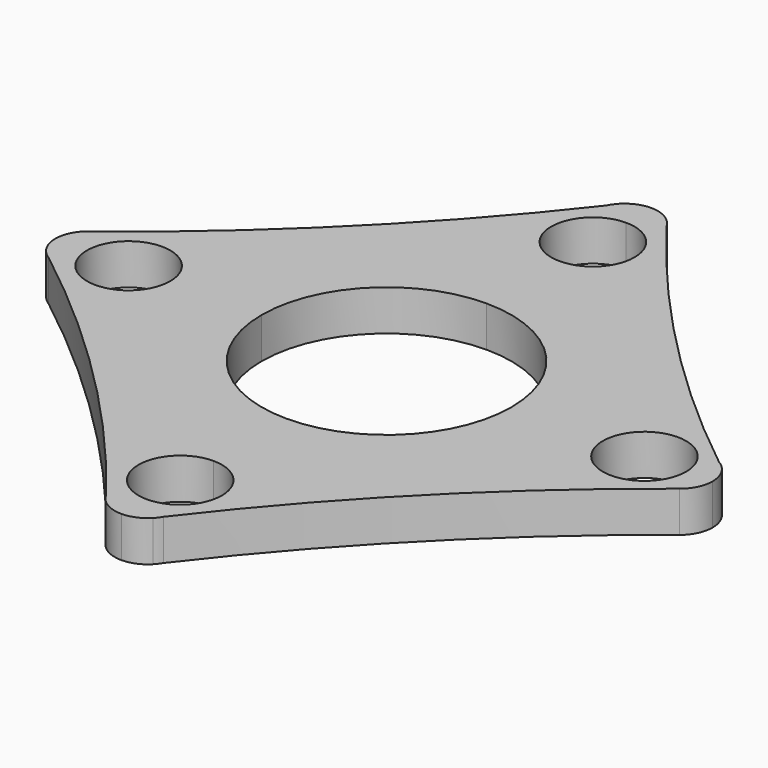
from build123d import *

# Parameters (mm, degrees)
F1_DEPTH = 1.5


with BuildPart() as f1:
    # F0 (on Top) → F1 (new body)
    with BuildSketch(Plane.XY):
        with BuildLine():
            ThreePointArc((-11.0335932724, 0), (-9.5, 1.5335932724), (-7.9664067276, 0))
            Line((-7.9664067276, 0), (-4.6, 0))
            ThreePointArc((-4.6, 0), (-3.2526911935, 3.2526911935), (0, 4.6))
            Line((0, 4.6), (0, 7.9664067276))
            ThreePointArc((0, 7.9664067276), (-1.5335932724, 9.5), (0, 11.0335932724))
            Line((0, 11.0335932724), (0, 12.2052515495))
            ThreePointArc((0, 12.2052515495), (-0.4345010394, 12.1317339839), (-0.8145803081, 11.9087188829))
            ThreePointArc((-0.8145803081, 11.9087188829), (-0.9635912872, 11.7146325201), (-1.1134019503, 11.5211627464))
            ThreePointArc((-1.1134019503, 11.5211627464), (-6.0214332546, 5.9647454006), (-11.5844815273, 1.064231252))
            ThreePointArc((-11.5844815273, 1.064231252), (-11.7185491453, 0.9605716693), (-11.8529124882, 0.8572956927))
            ThreePointArc((-11.8529124882, 0.8572956927), (-12.1114910997, 0.4629412091), (-12.2012897293, 0))
            Line((-12.2012897293, 0), (-11.0335932724, 0))
        make_face()
        with BuildLine():
            Line((-4.6, 0), (-7.9664067276, 0))
            ThreePointArc((-7.9664067276, 0), (-9.5, -1.5335932724), (-11.0335932724, 0))
            Line((-11.0335932724, 0), (-12.2012897293, 0))
            ThreePointArc((-12.2012897293, 0), (-12.1017179659, -0.4794729938), (-11.8217098669, -0.8812245989))
            ThreePointArc((-11.8217098669, -0.8812245989), (-11.721781237, -0.9580802015), (-11.6220162383, -1.0351480919))
            ThreePointArc((-11.6220162383, -1.0351480919), (-6.0202525949, -5.9659244981), (-1.0822216309, -11.5612941984))
            ThreePointArc((-1.0822216309, -11.5612941984), (-0.9646757294, -11.7132260984), (-0.8476226636, -11.8655380184))
            ThreePointArc((-0.8476226636, -11.8655380184), (-0.4559625925, -12.1137220892), (0, -12.1979305118))
            Line((0, -12.1979305118), (0, -11.0335932724))
            ThreePointArc((0, -11.0335932724), (-1.5335932724, -9.5), (0, -7.9664067276))
            Line((0, -7.9664067276), (0, -4.6))
            ThreePointArc((0, -4.6), (-3.2526911935, -3.2526911935), (-4.6, 0))
        make_face()
        with BuildLine():
            Line((0, 7.9664067276), (0, 4.6))
            ThreePointArc((0, 4.6), (3.2526911935, 3.2526911935), (4.6, 0))
            Line((4.6, 0), (7.9664067276, 0))
            ThreePointArc((7.9664067276, 0), (9.5, 1.5335932724), (11.0335932724, 0))
            Line((11.0335932724, 0), (12.0049398392, 0))
            ThreePointArc((12.0049398392, 0), (11.9193137164, 0.4573515512), (11.6687643937, 0.849432297))
            ThreePointArc((11.6687643937, 0.849432297), (11.5305346329, 0.9577272788), (11.3926261985, 1.0664311591))
            ThreePointArc((11.3926261985, 1.0664311591), (5.8870136821, 6.0076850195), (1.0395559509, 11.5960579882))
            ThreePointArc((1.0395559509, 11.5960579882), (0.9473724033, 11.7171151321), (0.8554998188, 11.838408441))
            ThreePointArc((0.8554998188, 11.838408441), (0.4640913385, 12.1065803567), (0, 12.2052515495))
            Line((0, 12.2052515495), (0, 11.0335932724))
            ThreePointArc((0, 11.0335932724), (1.0844142025, 10.5844142025), (1.5335932724, 9.5))
            ThreePointArc((1.5335932724, 9.5), (1.0844142025, 8.4155857975), (0, 7.9664067276))
        make_face()
        with BuildLine():
            ThreePointArc((4.6, 0), (3.2526911935, -3.2526911935), (0, -4.6))
            Line((0, -4.6), (0, -7.9664067276))
            ThreePointArc((0, -7.9664067276), (1.0844142025, -8.4155857975), (1.5335932724, -9.5))
            ThreePointArc((1.5335932724, -9.5), (1.0844142025, -10.5844142025), (0, -11.0335932724))
            Line((0, -11.0335932724), (0, -12.1979305118))
            ThreePointArc((0, -12.1979305118), (0.4647348704, -12.1017306528), (0.8576533678, -11.8355578385))
            ThreePointArc((0.8576533678, -11.8355578385), (0.9532380505, -11.7093930262), (1.0491591917, -11.5834838282))
            ThreePointArc((1.0491591917, -11.5834838282), (5.9633685423, -5.9301704288), (11.5511297333, -0.9415502985))
            ThreePointArc((11.5511297333, -0.9415502985), (11.8839118623, -0.5218059727), (12.0049398392, 0))
            Line((12.0049398392, 0), (11.0335932724, 0))
            ThreePointArc((11.0335932724, 0), (9.5, -1.5335932724), (7.9664067276, 0))
            Line((7.9664067276, 0), (4.6, 0))
        make_face()
        with BuildLine():
            ThreePointArc((-11.5844815273, 1.064231252), (-11.7259145151, 0.970125819), (-11.8529124882, 0.8572956927))
            ThreePointArc((-11.8529124882, 0.8572956927), (-11.7185491453, 0.9605716693), (-11.5844815273, 1.064231252))
        make_face()
        with BuildLine():
            ThreePointArc((-11.6220162383, -1.0351480919), (-11.721781237, -0.9580802015), (-11.8217098669, -0.8812245989))
            ThreePointArc((-11.8217098669, -0.8812245989), (-11.7258479783, -0.9633562144), (-11.6220162383, -1.0351480919))
        make_face()
        with BuildLine():
            ThreePointArc((-0.8145803081, 11.9087188829), (-0.9836129307, 11.7300700266), (-1.1134019503, 11.5211627464))
            ThreePointArc((-1.1134019503, 11.5211627464), (-0.9635912872, 11.7146325201), (-0.8145803081, 11.9087188829))
        make_face()
        with BuildLine():
            ThreePointArc((-0.8476226636, -11.8655380184), (-0.9646757294, -11.7132260984), (-1.0822216309, -11.5612941984))
            ThreePointArc((-1.0822216309, -11.5612941984), (-0.9769671574, -11.7227038795), (-0.8476226636, -11.8655380184))
        make_face()
        with BuildLine():
            ThreePointArc((1.0395559509, 11.5960579882), (0.9551101208, 11.72299164), (0.8554998188, 11.838408441))
            ThreePointArc((0.8554998188, 11.838408441), (0.9473724033, 11.7171151321), (1.0395559509, 11.5960579882))
        make_face()
        with BuildLine():
            ThreePointArc((1.0491591917, -11.5834838282), (0.9532380505, -11.7093930262), (0.8576533678, -11.8355578385))
            ThreePointArc((0.8576533678, -11.8355578385), (0.9616128176, -11.7157555094), (1.0491591917, -11.5834838282))
        make_face()
        with BuildLine():
            ThreePointArc((11.3926261985, 1.0664311591), (11.5305346329, 0.9577272788), (11.6687643937, 0.849432297))
            ThreePointArc((11.6687643937, 0.849432297), (11.5385404595, 0.9679149567), (11.3926261985, 1.0664311591))
        make_face()
    extrude(amount=F1_DEPTH)


solid = f1.part
